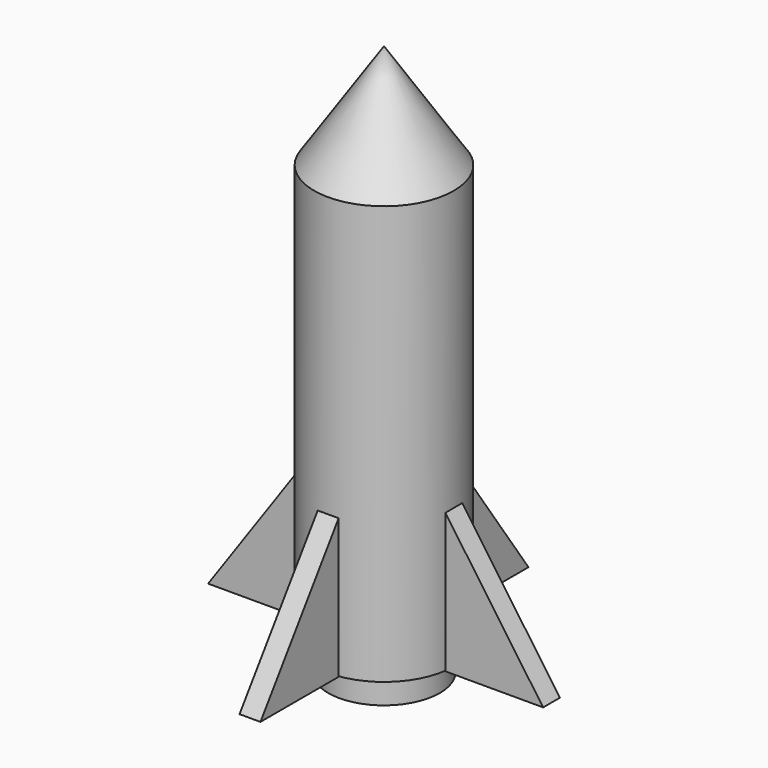
from build123d import *

# Parameters (mm, degrees)
F0_R      = 50
F1_DEPTH  = 300
F4_R      = 40
F5_DEPTH  = 20
F7_DEPTH  = 7.5
F8_ANGLE  = 90
F9_ANGLE  = -90
F10_ANGLE = 180


with BuildPart() as f1:
    # F0 (on Top) → F1 (new body)
    with BuildSketch(Plane.XY):
        Circle(F0_R)
    extrude(amount=-F1_DEPTH)

    # F2 (on Front) → F3 (revolve)
    with BuildSketch(Plane.XZ):
        Polygon((0, 75), (0, 0), (50, 0), align=None)
    revolve(axis=Axis((0, 0, 37.5), (0, 0, 1)))

    # F4 (on face) → F5 (join)
    with BuildSketch(Plane(origin=(0, 0, -300), x_dir=(1, 0, 0), z_dir=(0, 0, -1))):
        Circle(F4_R)
    extrude(amount=F5_DEPTH)


with BuildPart() as f7:
    # F6 (on Right) → F7 (new body, symmetric)
    with BuildSketch(Plane.YZ):
        Polygon((120, -300), (50, -200), (50, -300), align=None)
    extrude(amount=F7_DEPTH, both=True)


with BuildPart() as f8_1:
    # F8: copy of F7
    add(f7.part.rotate(Axis((0, 0, 0), (0, 0, 1)), F8_ANGLE))


with BuildPart() as f9_1:
    # F9: copy of F7
    add(f7.part.rotate(Axis((0, 0, 0), (0, 0, 1)), F9_ANGLE))


with BuildPart() as f10_1:
    # F10: copy of F7
    add(f7.part.rotate(Axis((0, 0, 0), (0, 0, 1)), F10_ANGLE))


solid = Compound([f1.part, f7.part, f8_1.part, f9_1.part, f10_1.part])
